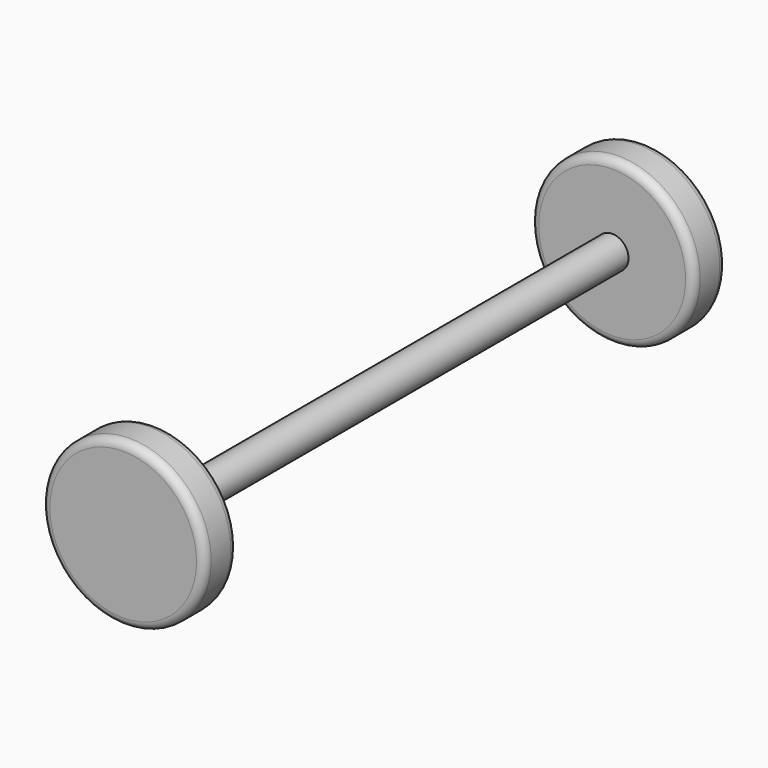
from build123d import *

# Parameters (mm, degrees)
F0_R     = 2
F1_DEPTH = 70
F2_R     = 10
F3_DEPTH = 5
F4_R     = 1
F5_R     = 10
F5_R_2   = 2
F6_DEPTH = 5
F7_R     = 1


# Not quite as in the source:
# - a feature names something its author has since deleted; it is built from what else it names


with BuildPart() as f1:
    # F0 (on Front) → F1 (new body)
    with BuildSketch(Plane.XZ):
        Circle(F0_R)
    extrude(amount=F1_DEPTH)

    # F2 (on face) → F3 (join)
    with BuildSketch(Plane.XZ.offset(70)):
        Circle(F2_R)
    extrude(amount=F3_DEPTH)

    # F4
    f4_edges = [f1.edges().sort_by_distance(p)[0] for p in [
        (-10, -70, 0),
        (-10, -75, 0),
    ]]
    fillet(f4_edges, radius=F4_R)

    # F5 (on face) → F6 (join)
    with BuildSketch(Plane(origin=(0, 0, 0), x_dir=(-1, 0, 0), z_dir=(0, 1, 0))):
        Circle(F5_R)
        Circle(F5_R_2, mode=Mode.SUBTRACT)
        Circle(F5_R_2)
    extrude(amount=F6_DEPTH)

    # F7
    f7_edges = [f1.edges().sort_by_distance(p)[0] for p in [
        (10, 0, 0),
        (10, 5, 0),
    ]]
    fillet(f7_edges, radius=F7_R)


solid = f1.part
